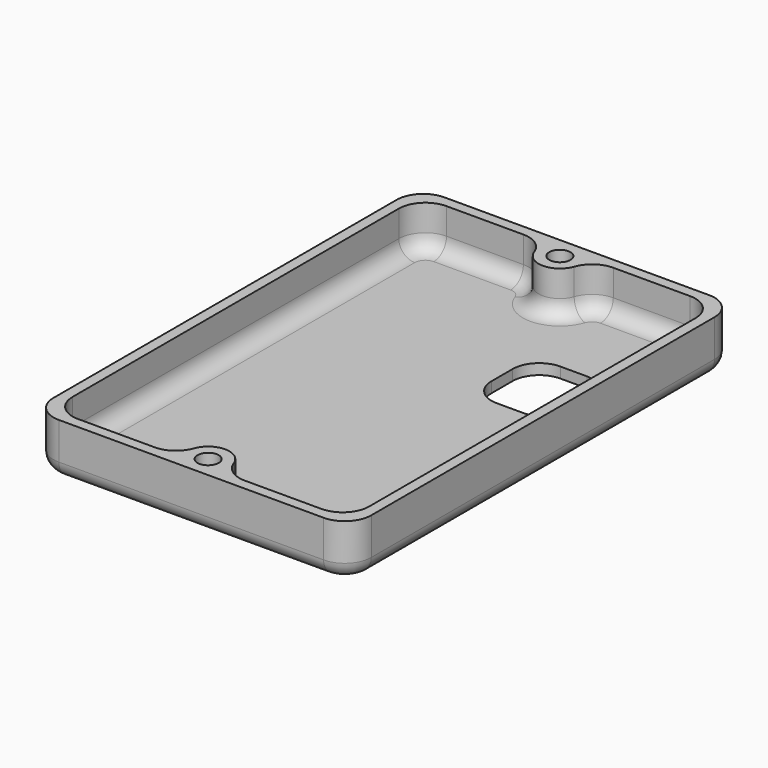
from build123d import *

# Parameters (mm, degrees)
F3_W          = 60
F3_H          = 91
F4_DEPTH      = 10
F5_W          = 56
F5_H          = 87
F6_DEPTH      = 8
F7_R          = 4
F8_DEPTH      = 10
F9_R          = 2
F10_DEPTH     = 10.001
F11_R         = 5
F12_R         = 5
F13_T1_DEPTH  = 77
F13_T3_DEPTH  = 14.5147186258
F13_T5_DEPTH  = 14.5147186258
F13_T8_ANGLE  = 90
F13_T10_ANGLE = 70.5287793655
F13_T12_ANGLE = 141.057558731
F13_T14_ANGLE = 90
F13_T16_ANGLE = 70.5287793655
F13_T18_ANGLE = 70.5287793655
F13_T20_ANGLE = 90
F13_T22_ANGLE = 141.057558731
F13_T24_ANGLE = 70.5287793655
F13_T26_ANGLE = 90
F13_T27_DEPTH = 81
F13_T29_DEPTH = 50
F13_T32_ANGLE = 90
F13_T34_ANGLE = 90
F13_T36_ANGLE = 90
F13_T38_ANGLE = 90
F14_W         = 15
F14_H         = 15
F15_DEPTH     = 2.0010001
F16_R         = 5


# Not quite as in the source:
# - a fillet or chamfer that OpenCascade refuses, or shapes differently, is made with other operations: its cross-section is extruded or revolved along the edge and cut away or added


with BuildPart() as f4:
    # F3 (on Top) → F4 (new body)
    with BuildSketch(Plane.XY):
        Rectangle(F3_W, F3_H)
    extrude(amount=F4_DEPTH)

    # F5 (on face) → F6 (cut)
    with BuildSketch(Plane.XY.offset(10)):
        Rectangle(F5_W, F5_H)
    extrude(amount=-F6_DEPTH, mode=Mode.SUBTRACT)

    # F7 (on face) → F8 (join)
    with BuildSketch(Plane(origin=(0, 0, 0), x_dir=(1, 0, 0), z_dir=(0, 0, -1))):
        with Locations((0, -41.5)):
            Circle(F7_R)
        with Locations((0, 41.5)):
            Circle(F7_R)
    extrude(amount=-F8_DEPTH)

    # F9 (on face) → F10 (cut, through all)
    with BuildSketch(Plane(origin=(0, 0, 0), x_dir=(1, 0, 0), z_dir=(0, 0, -1))):
        with Locations((0, -41.5)):
            Circle(F9_R)
        with Locations((0, 41.5)):
            Circle(F9_R)
    extrude(amount=-F10_DEPTH, mode=Mode.SUBTRACT)

    # F11
    f11_edges = [f4.edges().sort_by_distance(p)[0] for p in [
        (3.464102, 43.5, 6),
        (-3.464102, 43.5, 6),
        (-3.464102, -43.5, 6),
        (3.464102, -43.5, 6),
    ]]
    fillet(f11_edges, radius=F11_R)

    # F12
    f12_edges = [f4.edges().sort_by_distance(p)[0] for p in [
        (30, -45.5, 5),
        (-30, -45.5, 5),
        (30, 45.5, 5),
        (-30, 45.5, 5),
        (28, -43.5, 6),
        (-28, -43.5, 6),
        (-28, 43.5, 6),
        (28, 43.5, 6),
    ]]
    fillet(f12_edges, radius=F12_R)

    # F13: fillet of radius 3 on 24 edges, made by hand

    # F13_s2 → F13_t1 (join)
    with BuildSketch(Plane.XZ.offset(-38.5)):
        with BuildLine():
            ThreePointArc((-28, 5), (-27.1213203436, 2.8786796564), (-25, 2))
            Line((-25, 2), (-28, 2))
            Line((-28, 2), (-28, 5))
        make_face()
        with BuildLine():
            ThreePointArc((28, 5), (27.1213203436, 2.8786796564), (25, 2))
            Line((25, 2), (28, 2))
            Line((28, 2), (28, 5))
        make_face()
    extrude(amount=F13_T1_DEPTH)

    # F13_s4 → F13_t3 (join)
    with BuildSketch(Plane.YZ.offset(8.4852813742)):
        with BuildLine():
            ThreePointArc((-43.5, 5), (-42.6213203436, 2.8786796564), (-40.5, 2))
            Line((-40.5, 2), (-43.5, 2))
            Line((-43.5, 2), (-43.5, 5))
        make_face()
        with BuildLine():
            ThreePointArc((43.5, 5), (42.6213203436, 2.8786796564), (40.5, 2))
            Line((40.5, 2), (43.5, 2))
            Line((43.5, 2), (43.5, 5))
        make_face()
    extrude(amount=F13_T3_DEPTH)

    # F13_s6 → F13_t5 (join)
    with BuildSketch(Plane.YZ.offset(-23)):
        with BuildLine():
            ThreePointArc((-43.5, 5), (-42.6213203436, 2.8786796564), (-40.5, 2))
            Line((-40.5, 2), (-43.5, 2))
            Line((-43.5, 2), (-43.5, 5))
        make_face()
        with BuildLine():
            ThreePointArc((43.5, 5), (42.6213203436, 2.8786796564), (40.5, 2))
            Line((40.5, 2), (43.5, 2))
            Line((43.5, 2), (43.5, 5))
        make_face()
    extrude(amount=F13_T5_DEPTH)

    # F13_s7 → F13_t8 (revolve)
    with BuildSketch(Plane.YZ.offset(23)):
        with BuildLine():
            ThreePointArc((-43.5, 5), (-42.6213203436, 2.8786796564), (-40.5, 2))
            Line((-40.5, 2), (-43.5, 2))
            Line((-43.5, 2), (-43.5, 5))
        make_face()
    revolve(axis=Axis((23, -38.5, 2), (0, 0, 1)), revolution_arc=F13_T8_ANGLE)

    # F13_s9 → F13_t10 (revolve)
    with BuildSketch(Plane.YZ.offset(8.4852813742)):
        with BuildLine():
            ThreePointArc((-43.5, 5), (-42.6213203436, 2.8786796564), (-40.5, 2))
            Line((-40.5, 2), (-43.5, 2))
            Line((-43.5, 2), (-43.5, 5))
        make_face()
    revolve(axis=Axis((8.4852813742, -38.5, 2), (0, 0, -1)), revolution_arc=F13_T10_ANGLE)

    # F13_s11 → F13_t12 (revolve)
    with BuildSketch(Plane(origin=(-13.0421917419, -36.8888888889, 0), x_dir=(0, 0, 1), z_dir=(-0.3333333333, -0.9428090416, 0))):
        with BuildLine():
            ThreePointArc((5, -9.8333333333), (2.8786796564, -8.9546536769), (2, -6.8333333333))
            Line((2, -6.8333333333), (2, -9.8333333333))
            Line((2, -9.8333333333), (5, -9.8333333333))
        make_face()
    revolve(axis=Axis((0, -41.5, 2), (0, 0, -1)), revolution_arc=F13_T12_ANGLE)

    # F13_s13 → F13_t14 (revolve)
    with BuildSketch(Plane.XZ.offset(-38.5)):
        with BuildLine():
            ThreePointArc((28, 5), (27.1213203436, 2.8786796564), (25, 2))
            Line((25, 2), (28, 2))
            Line((28, 2), (28, 5))
        make_face()
    revolve(axis=Axis((23, 38.5, 2), (0, 0, 1)), revolution_arc=F13_T14_ANGLE)

    # F13_s15 → F13_t16 (revolve)
    with BuildSketch(Plane(origin=(-13.0421917419, -36.8888888889, 0), x_dir=(0, 0, 1), z_dir=(0.3333333333, 0.9428090416, 0))):
        with BuildLine():
            ThreePointArc((5, 9.8333333333), (2.8786796564, 8.9546536769), (2, 6.8333333333))
            Line((2, 6.8333333333), (2, 9.8333333333))
            Line((2, 9.8333333333), (5, 9.8333333333))
        make_face()
    revolve(axis=Axis((-8.4852813742, -38.5, 2), (0, 0, -1)), revolution_arc=F13_T16_ANGLE)

    # F13_s17 → F13_t18 (revolve)
    with BuildSketch(Plane.YZ.offset(8.4852813742)):
        with BuildLine():
            ThreePointArc((43.5, 5), (42.6213203436, 2.8786796564), (40.5, 2))
            Line((40.5, 2), (43.5, 2))
            Line((43.5, 2), (43.5, 5))
        make_face()
    revolve(axis=Axis((8.4852813742, 38.5, 2), (0, 0, 1)), revolution_arc=F13_T18_ANGLE)

    # F13_s19 → F13_t20 (revolve)
    with BuildSketch(Plane.YZ.offset(-23)):
        with BuildLine():
            ThreePointArc((-43.5, 5), (-42.6213203436, 2.8786796564), (-40.5, 2))
            Line((-40.5, 2), (-43.5, 2))
            Line((-43.5, 2), (-43.5, 5))
        make_face()
    revolve(axis=Axis((-23, -38.5, 2), (0, 0, -1)), revolution_arc=F13_T20_ANGLE)

    # F13_s21 → F13_t22 (revolve)
    with BuildSketch(Plane(origin=(13.0421917419, 36.8888888889, 0), x_dir=(0, 0, 1), z_dir=(0.3333333333, 0.9428090416, 0))):
        with BuildLine():
            ThreePointArc((5, -9.8333333333), (2.8786796564, -8.9546536769), (2, -6.8333333333))
            Line((2, -6.8333333333), (2, -9.8333333333))
            Line((2, -9.8333333333), (5, -9.8333333333))
        make_face()
    revolve(axis=Axis((0, 41.5, 2), (0, 0, -1)), revolution_arc=F13_T22_ANGLE)

    # F13_s23 → F13_t24 (revolve)
    with BuildSketch(Plane(origin=(-13.0421917419, 36.8888888889, 0), x_dir=(0, 0, 1), z_dir=(0.3333333333, -0.9428090416, 0))):
        with BuildLine():
            ThreePointArc((5, -9.8333333333), (2.8786796564, -8.9546536769), (2, -6.8333333333))
            Line((2, -6.8333333333), (2, -9.8333333333))
            Line((2, -9.8333333333), (5, -9.8333333333))
        make_face()
    revolve(axis=Axis((-8.4852813742, 38.5, 2), (0, 0, 1)), revolution_arc=F13_T24_ANGLE)

    # F13_s25 → F13_t26 (revolve)
    with BuildSketch(Plane.XZ.offset(-38.5)):
        with BuildLine():
            ThreePointArc((-28, 5), (-27.1213203436, 2.8786796564), (-25, 2))
            Line((-25, 2), (-28, 2))
            Line((-28, 2), (-28, 5))
        make_face()
    revolve(axis=Axis((-23, 38.5, 2), (0, 0, -1)), revolution_arc=F13_T26_ANGLE)

    # F13_s28 → F13_t27 (cut)
    with BuildSketch(Plane.XZ.offset(-40.5)):
        with BuildLine():
            ThreePointArc((30, 3), (29.1213203436, 0.8786796564), (27, 0))
            Line((27, 0), (30, 0))
            Line((30, 0), (30, 3))
        make_face()
        with BuildLine():
            ThreePointArc((-30, 3), (-29.1213203436, 0.8786796564), (-27, 0))
            Line((-27, 0), (-30, 0))
            Line((-30, 0), (-30, 3))
        make_face()
    extrude(amount=F13_T27_DEPTH, mode=Mode.SUBTRACT)

    # F13_s30 → F13_t29 (cut)
    with BuildSketch(Plane.YZ.offset(-25)):
        with BuildLine():
            ThreePointArc((-45.5, 3), (-44.6213203436, 0.8786796564), (-42.5, 0))
            Line((-42.5, 0), (-45.5, 0))
            Line((-45.5, 0), (-45.5, 3))
        make_face()
        with BuildLine():
            ThreePointArc((45.5, 3), (44.6213203436, 0.8786796564), (42.5, 0))
            Line((42.5, 0), (45.5, 0))
            Line((45.5, 0), (45.5, 3))
        make_face()
    extrude(amount=F13_T29_DEPTH, mode=Mode.SUBTRACT)

    # F13_s31 → F13_t32 (revolve, cut)
    with BuildSketch(Plane.YZ.offset(25)):
        with BuildLine():
            ThreePointArc((-45.5, 3), (-44.6213203436, 0.8786796564), (-42.5, 0))
            Line((-42.5, 0), (-45.5, 0))
            Line((-45.5, 0), (-45.5, 3))
        make_face()
    revolve(axis=Axis((25, -40.5, 0), (0, 0, 1)), revolution_arc=F13_T32_ANGLE, mode=Mode.SUBTRACT)

    # F13_s33 → F13_t34 (revolve, cut)
    with BuildSketch(Plane.YZ.offset(-25)):
        with BuildLine():
            ThreePointArc((-45.5, 3), (-44.6213203436, 0.8786796564), (-42.5, 0))
            Line((-42.5, 0), (-45.5, 0))
            Line((-45.5, 0), (-45.5, 3))
        make_face()
    revolve(axis=Axis((-25, -40.5, 0), (0, 0, -1)), revolution_arc=F13_T34_ANGLE, mode=Mode.SUBTRACT)

    # F13_s35 → F13_t36 (revolve, cut)
    with BuildSketch(Plane.XZ.offset(-40.5)):
        with BuildLine():
            ThreePointArc((30, 3), (29.1213203436, 0.8786796564), (27, 0))
            Line((27, 0), (30, 0))
            Line((30, 0), (30, 3))
        make_face()
    revolve(axis=Axis((25, 40.5, 0), (0, 0, 1)), revolution_arc=F13_T36_ANGLE, mode=Mode.SUBTRACT)

    # F13_s37 → F13_t38 (revolve, cut)
    with BuildSketch(Plane.XZ.offset(-40.5)):
        with BuildLine():
            ThreePointArc((-30, 3), (-29.1213203436, 0.8786796564), (-27, 0))
            Line((-27, 0), (-30, 0))
            Line((-30, 0), (-30, 3))
        make_face()
    revolve(axis=Axis((-25, 40.5, 0), (0, 0, -1)), revolution_arc=F13_T38_ANGLE, mode=Mode.SUBTRACT)

    # F14 (on face) → F15 (cut, through all)
    with BuildSketch(Plane.XY.offset(2)):
        with Locations((15, 18.5)):
            Rectangle(F14_W, F14_H)
    extrude(amount=-F15_DEPTH, mode=Mode.SUBTRACT)

    # F16
    f16_edges = [f4.edges().sort_by_distance(p)[0] for p in [
        (7.5, 26, 1),
        (22.5, 26, 1),
        (22.5, 11, 1),
        (7.5, 11, 1),
    ]]
    fillet(f16_edges, radius=F16_R)


solid = f4.part
